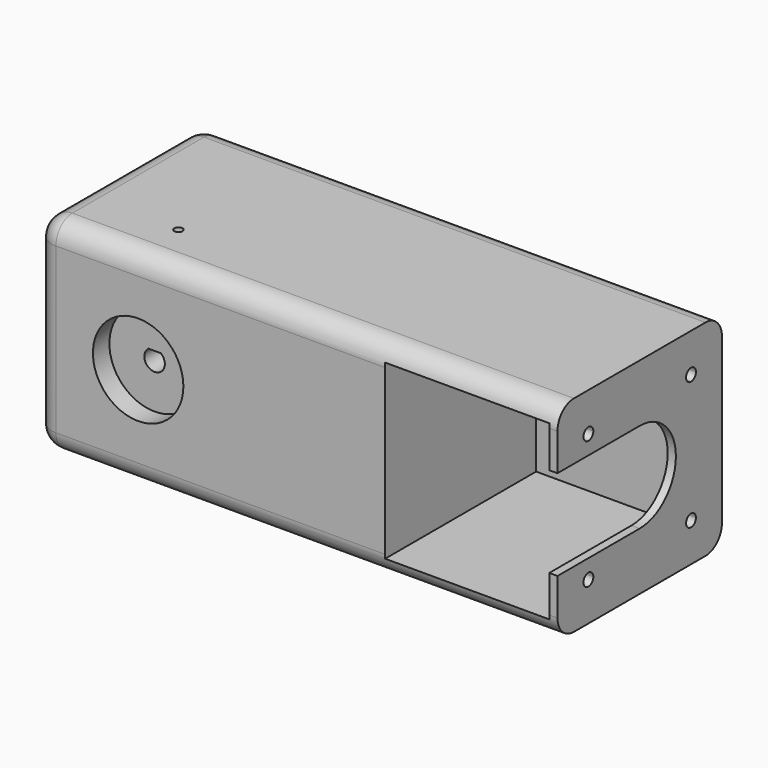
from build123d import *

# Parameters (mm, degrees)
F0_W           = 127
F0_H           = 50
F1_DEPTH       = 50
F3_DEPTH       = 42
F4_R           = 11
F5_DEPTH       = 5
F7_DEPTH       = 15
F8_T2_ANGLE    = 343.7894292622
F9_R           = 5
F12_W          = 40
F12_H          = 42
F13_DEPTH      = 46
F14_R          = 1.6
F15_DEPTH      = 1
F16_R          = 1
F17_DEPTH      = 2
F17_DEPTH_BACK = 1.03
F18_DEPTH      = 25
F19_DEPTH      = 2
F20_DEPTH      = 25


# Not quite as in the source:
# - a fillet or chamfer that OpenCascade refuses, or shapes differently, is made with other operations: its cross-section is extruded or revolved along the edge and cut away or added


with BuildPart() as f1:
    # F0 (on Front) → F1 (new body)
    with BuildSketch(Plane.XZ):
        Rectangle(F0_W, F0_H)
    extrude(amount=F1_DEPTH)

    # F2 (on face) → F3 (cut)
    with BuildSketch(Plane.YZ.offset(63.5)):
        Polygon((-41.7573593129, 21), (-46, 16.7573593129), (-46, -16.7573593129), (-41.7573593129, -21), (-8.2426406871, -21), (-4, -16.7573593129), (-4, 16.7573593129), (-8.2426406871, 21), align=None)
    extrude(amount=-F3_DEPTH, mode=Mode.SUBTRACT)

    # F4 (on face) → F5 (cut)
    with BuildSketch(Plane.XZ.offset(50)):
        with Locations((-38.5, 0)):
            Circle(F4_R)
    extrude(amount=-F5_DEPTH, mode=Mode.SUBTRACT)

    # F6 (on face) → F7 (cut)
    with BuildSketch(Plane.XZ.offset(45)):
        with BuildLine():
            Line((-37, 2), (-40, 2))
            ThreePointArc((-40, 2), (-38.5, -2.5), (-37, 2))
        make_face()
    extrude(amount=-F7_DEPTH, mode=Mode.SUBTRACT)

    # F8: fillet of radius 0.5 on 1 edges, made by hand

    # F8_s1 → F8_t2 (revolve)
    with BuildSketch(Plane(origin=(-37.7346622942, 0, -5.3739891953), x_dir=(0, 1, 0), z_dir=(0.9900106558, 0, 0.1409925581))):
        with BuildLine():
            ThreePointArc((-30.5, 7.9282134883), (-30.1464466094, 7.7817668789), (-30, 7.4282134883))
            Line((-30, 7.4282134883), (-30, 7.9282134883))
            Line((-30, 7.9282134883), (-30.5, 7.9282134883))
        make_face()
    revolve(axis=Axis((-38.5, -30, 0), (0, -1, 0)), revolution_arc=F8_T2_ANGLE)

    # F9
    f9_edges = [f1.edges().sort_by_distance(p)[0] for p in [
        (0, -50, 25),
        (0, -50, -25),
        (0, 0, 25),
        (0, 0, -25),
        (-63.5, -25, 25),
        (-63.5, -25, -25),
        (-63.5, 0, 0),
        (-63.5, -50, 0),
    ]]
    fillet(f9_edges, radius=F9_R)

    # F12 (on face) → F13 (cut)
    with BuildSketch(Plane.XZ.offset(50)):
        with Locations((41.5, 0)):
            Rectangle(F12_W, F12_H)
    extrude(amount=-F13_DEPTH, mode=Mode.SUBTRACT)

    # F14 (on face) → F15 (cut)
    with BuildSketch(Plane(origin=(0, 0, 0), x_dir=(-1, 0, 0), z_dir=(0, 1, 0))):
        with Locations((-46.0031795697, -4.1205275279)):
            Circle(F14_R)
        with Locations((-22.6282365388, 5.5031795697)):
            Circle(F14_R)
    extrude(amount=-F15_DEPTH, mode=Mode.SUBTRACT)

    # F16 (on face) → F17 (cut, two sides)
    with BuildSketch(Plane(origin=(0, 0, 2), x_dir=(1, 0, 0), z_dir=(0, 0, -1))) as f17_sk:
        Polygon((-36.5, 38.9047005384), (-38.5, 40.0594010768), (-40.5, 38.9047005384), (-40.5, 36.5952994616), (-38.5, 35.4405989232), (-36.5, 36.5952994616), align=None)
        with Locations((-38.5, 37.75)):
            Circle(F16_R, mode=Mode.SUBTRACT)
    extrude(amount=-F17_DEPTH, mode=Mode.SUBTRACT)
    extrude(f17_sk.sketch, amount=F17_DEPTH_BACK, mode=Mode.SUBTRACT)

    # F18 (cut): a face of the model
    f18_faces = [f1.faces().sort_by_distance(p)[0] for p in [
        (-38.5, -37.75, 2),
    ]]
    extrude(f18_faces, amount=-F18_DEPTH, mode=Mode.SUBTRACT)

    # F10 (on face) → F19 (join)
    with BuildSketch(Plane.YZ.offset(63.5)):
        Polygon((-46, 16.7573593129), (-46, -16.7573593129), (-41.7573593129, -21), (-8.2426406871, -21), (-4, -16.7573593129), (-4, 16.7573593129), (-8.2426406871, 21), (-16.9, 21), (-33.1, 21), (-41.7573593129, 21), align=None)
        with BuildLine():
            Line((-10.9, -15.6), (-39.1, -15.6))
            ThreePointArc((-39.1, -15.6), (-41.6606601718, -16.6606601718), (-40.6, -14.1))
            Line((-40.6, -14.1), (-40.6, 14.1))
            ThreePointArc((-40.6, 14.1), (-41.6606601718, 16.6606601718), (-39.1, 15.6))
            Line((-39.1, 15.6), (-10.9, 15.6))
            ThreePointArc((-10.9, 15.6), (-9.4, 17.1), (-7.9, 15.6))
            ThreePointArc((-7.9, 15.6), (-8.3393398282, 14.5393398282), (-9.4, 14.1))
            Line((-9.4, 14.1), (-9.4, -14.1))
            ThreePointArc((-9.4, -14.1), (-8.3393398282, -14.5393398282), (-7.9, -15.6))
            ThreePointArc((-7.9, -15.6), (-9.4, -17.1), (-10.9, -15.6))
        make_face(mode=Mode.SUBTRACT)
        with BuildLine():
            ThreePointArc((-40.6, -14.1), (-39.5393398282, -14.5393398282), (-39.1, -15.6))
            Line((-39.1, -15.6), (-10.9, -15.6))
            ThreePointArc((-10.9, -15.6), (-10.4606601718, -14.5393398282), (-9.4, -14.1))
            Line((-9.4, -14.1), (-9.4, 14.1))
            ThreePointArc((-9.4, 14.1), (-10.4606601718, 14.5393398282), (-10.9, 15.6))
            Line((-10.9, 15.6), (-39.1, 15.6))
            ThreePointArc((-39.1, 15.6), (-39.5393398282, 14.5393398282), (-40.6, 14.1))
            Line((-40.6, 14.1), (-40.6, -14.1))
        make_face()
    extrude(amount=-F19_DEPTH)

    # F11 (on face) → F20 (cut)
    with BuildSketch(Plane.YZ.offset(63.5)):
        with BuildLine():
            Line((-50, -11), (-25, -11))
            ThreePointArc((-25, -11), (-14, 0), (-25, 11))
            Line((-25, 11), (-50, 11))
            Line((-50, 11), (-50, -11))
        make_face()
    extrude(amount=-F20_DEPTH, mode=Mode.SUBTRACT)


solid = f1.part
